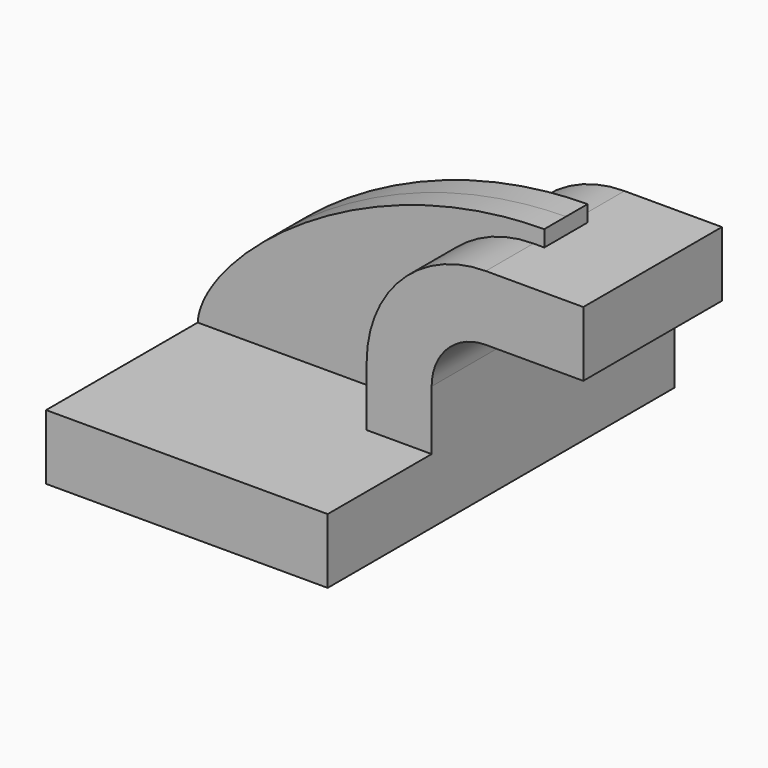
from build123d import *

# Parameters (mm, degrees)
F1_DEPTH = 63.5
F0_W     = 25.4
F0_H     = 19.05
F2_DEPTH = 25.4
F3_DEPTH = 7.9375


# Not quite as in the source:
# - a feature of the source that left no trace in its solid (it failed there, or was rolled back) is left out


with BuildPart() as f1:
    # F0 (on Front) → F1 (new body, symmetric)
    with BuildSketch(Plane.XZ):
        Polygon((-41.275, -9.525), (41.275, -9.525), (41.275, 9.525), (22.225, 9.525), (-41.275, 9.525), align=None)
    extrude(amount=F1_DEPTH, both=True)

    # F0 (on Front) → F2 (join, symmetric)
    with BuildSketch(Plane.XZ):
        with BuildLine():
            Line((22.225, 9.525), (41.275, 9.525))
            Line((41.275, 9.525), (41.275, 27.0002))
            ThreePointArc((41.275, 27.0002), (45.9246798487, 38.2255201513), (57.15, 42.8752))
            Line((57.15, 42.8752), (60.325, 42.8752))
            Line((60.325, 42.8752), (60.325, 61.9252))
            Line((60.325, 61.9252), (57.15, 61.9252))
            ThreePointArc((57.15, 61.9252), (32.4542956671, 51.6959043329), (22.225, 27.0002))
            Line((22.225, 27.0002), (22.225, 9.525))
        make_face()
        with Locations((73.025, 52.4002)):
            Rectangle(F0_W, F0_H)
    extrude(amount=F2_DEPTH, both=True)

    # F0 (on Front) → F3 (join, symmetric)
    with BuildSketch(Plane.XZ):
        with BuildLine():
            add(Edge.make_bspline(
                [(-41.275, 9.525), (-40.3944440186, 27.1777566522), (4.0625981055, 66.2999525666), (60.325, 66.675)],
                knots=[0, 0, 0, 0, 116.5705044169, 116.5705044169, 116.5705044169, 116.5705044169], degree=3))
            Line((-41.275, 9.525), (22.225, 9.525))
            Line((22.225, 9.525), (22.225, 27.0002))
            ThreePointArc((22.225, 27.0002), (32.4542956671, 51.6959043329), (57.15, 61.9252))
            Line((57.15, 61.9252), (60.325, 61.9252))
            Line((60.325, 61.9252), (60.325, 66.675))
        make_face()
    extrude(amount=F3_DEPTH, both=True)


solid = f1.part
